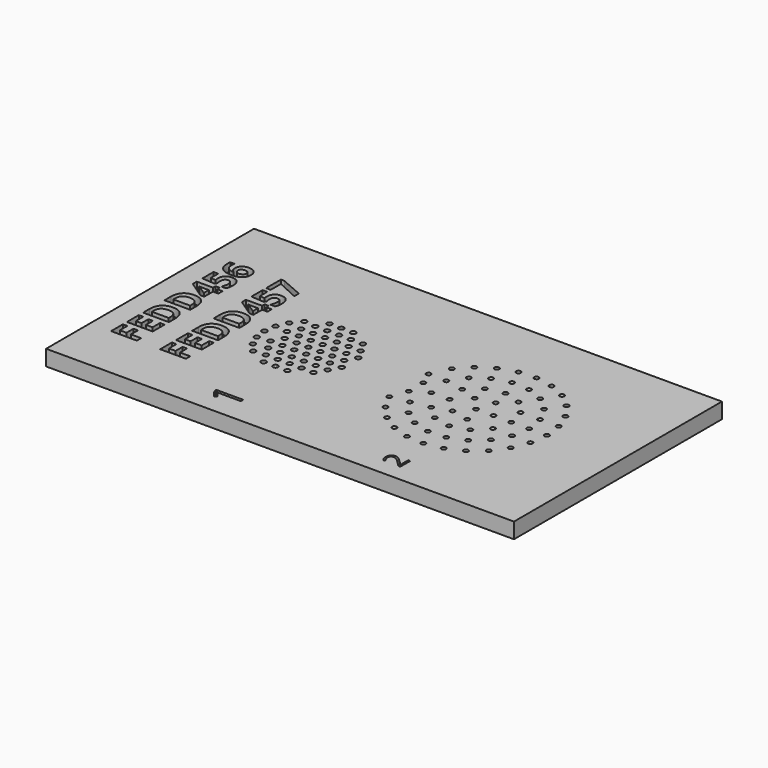
from build123d import *

# Parameters (mm, degrees)
F0_W           = 90
F0_H           = 50
F1_DEPTH       = 3
F2_TEXT_SIZE   = 6.9444444444
F2_TEXT_SIZE_2 = 7.24801812
F2_TEXT_SIZE_3 = 5.1460734388
F3_DEPTH       = 1.5
F4_R           = 0.5
F4_R_2         = 0.45
F5_DEPTH       = 3


# Not quite as in the source:
# - Text() gives the source's letters only with a copy of the font that has no kerning and outlines rounded to 1/6400 em; it was checked with that copy


with BuildPart() as f1:
    # F0 (on Top) → F1 (new body)
    with BuildSketch(Plane.XY):
        with Locations((1.8412768841, 3.3350909071)):
            Rectangle(F0_W, F0_H)
    extrude(amount=F1_DEPTH)

    # F2 (on face) → F3 (cut)
    with BuildSketch(Plane.XY.offset(3)):
        with Locations(Location((-34.1587231159, -11.7149090929), (0, 0, 90))):
            Text('FEDD456', F2_TEXT_SIZE, font='Open Sans', font_style=FontStyle.BOLD, text_align=(TextAlign.LEFT, TextAlign.BOTTOM))
        with Locations(Location((-24.7142786715, -11.7149090929), (0, 0, 90))):
            Text('FEDD457', F2_TEXT_SIZE, font='Open Sans', font_style=FontStyle.BOLD, text_align=(TextAlign.LEFT, TextAlign.BOTTOM))
        with Locations(Location((-9.6570708402, -18.6649090929), (0, 0, 90))):
            Text('1', F2_TEXT_SIZE_2, font='Open Sans', text_align=(TextAlign.LEFT, TextAlign.BOTTOM))
        with Locations(Location((22.3617675547, -18.6649090929), (0, 0, 90))):
            Text('2', F2_TEXT_SIZE_3, font='Open Sans', text_align=(TextAlign.LEFT, TextAlign.BOTTOM))
    extrude(amount=-F3_DEPTH, mode=Mode.SUBTRACT)

    # F4 (on face) → F5 (cut, through all)
    with BuildSketch(Plane.XY.offset(3)):
        with BuildLine():
            ThreePointArc((-20.6587231159, 3.3350909071), (-21.1587231159, 3.8350909071), (-21.6587231159, 3.3350909071))
            Line((-21.6587231159, 3.3350909071), (-20.6587231159, 3.3350909071))
        make_face()
        with BuildLine():
            ThreePointArc((-12.7987231159, 11.7449888556), (-13.1987231159, 11.2550909071), (-12.7987231159, 10.7651929585))
            Line((-12.7987231159, 10.7651929585), (-12.7987231159, 11.7449888556))
        make_face()
        with BuildLine():
            Line((-12.7987231159, 11.7449888556), (-12.7987231159, 10.7651929585))
            ThreePointArc((-12.7987231159, 10.7651929585), (-12.3824953499, 10.8677925724), (-12.1987231159, 11.2550909071))
            ThreePointArc((-12.1987231159, 11.2550909071), (-12.3824953499, 11.6423892417), (-12.7987231159, 11.7449888556))
        make_face()
        with BuildLine():
            ThreePointArc((-12.7987231159, 7.8049888556), (-13.1987231159, 7.3150909071), (-12.7987231159, 6.8251929585))
            Line((-12.7987231159, 6.8251929585), (-12.7987231159, 7.8049888556))
        make_face()
        with BuildLine():
            Line((-12.7987231159, 7.8049888556), (-12.7987231159, 6.8251929585))
            ThreePointArc((-12.7987231159, 6.8251929585), (-12.3824953499, 6.9277925724), (-12.1987231159, 7.3150909071))
            ThreePointArc((-12.1987231159, 7.3150909071), (-12.3824953499, 7.7023892417), (-12.7987231159, 7.8049888556))
        make_face()
        with BuildLine():
            ThreePointArc((-5.3387231159, 3.3350909071), (-5.8387231159, 3.8350909071), (-6.3387231159, 3.3350909071))
            Line((-6.3387231159, 3.3350909071), (-5.3387231159, 3.3350909071))
        make_face()
        with BuildLine():
            Line((-5.3387231159, 3.3350909071), (-6.3387231159, 3.3350909071))
            ThreePointArc((-6.3387231159, 3.3350909071), (-5.8387231159, 2.8350909071), (-5.3387231159, 3.3350909071))
        make_face()
        with BuildLine():
            ThreePointArc((-7.6287231159, 3.3350909071), (-8.1287231159, 3.8350909071), (-8.6287231159, 3.3350909071))
            Line((-8.6287231159, 3.3350909071), (-7.6287231159, 3.3350909071))
        make_face()
        with BuildLine():
            Line((-7.6287231159, 3.3350909071), (-8.6287231159, 3.3350909071))
            ThreePointArc((-8.6287231159, 3.3350909071), (-8.1287231159, 2.8350909071), (-7.6287231159, 3.3350909071))
        make_face()
        with BuildLine():
            ThreePointArc((-9.9087231159, 3.3350909071), (-10.4087231159, 3.8350909071), (-10.9087231159, 3.3350909071))
            Line((-10.9087231159, 3.3350909071), (-9.9087231159, 3.3350909071))
        make_face()
        with BuildLine():
            Line((-9.9087231159, 3.3350909071), (-10.9087231159, 3.3350909071))
            ThreePointArc((-10.9087231159, 3.3350909071), (-10.4087231159, 2.8350909071), (-9.9087231159, 3.3350909071))
        make_face()
        with BuildLine():
            ThreePointArc((-12.1987231159, -4.5849090929), (-12.3824953499, -4.1976107583), (-12.7987231159, -4.0950111444))
            Line((-12.7987231159, -4.0950111444), (-12.7987231159, -5.0748070415))
            ThreePointArc((-12.7987231159, -5.0748070415), (-12.3824953499, -4.9722074276), (-12.1987231159, -4.5849090929))
        make_face()
        with BuildLine():
            Line((-12.7987231159, -5.0748070415), (-12.7987231159, -4.0950111444))
            ThreePointArc((-12.7987231159, -4.0950111444), (-13.1987231159, -4.5849090929), (-12.7987231159, -5.0748070415))
        make_face()
        with BuildLine():
            ThreePointArc((-12.1987231159, -0.6449090929), (-12.3824953499, -0.2576107583), (-12.7987231159, -0.1550111444))
            Line((-12.7987231159, -0.1550111444), (-12.7987231159, -1.1348070415))
            ThreePointArc((-12.7987231159, -1.1348070415), (-12.3824953499, -1.0322074276), (-12.1987231159, -0.6449090929))
        make_face()
        with BuildLine():
            Line((-12.7987231159, -1.1348070415), (-12.7987231159, -0.1550111444))
            ThreePointArc((-12.7987231159, -0.1550111444), (-13.1987231159, -0.6449090929), (-12.7987231159, -1.1348070415))
        make_face()
        with BuildLine():
            ThreePointArc((-12.7987231159, 3.8249888556), (-13.0860214505, 3.6513186731), (-13.1987231159, 3.3350909071))
            Line((-13.1987231159, 3.3350909071), (-12.7987231159, 3.3350909071))
            Line((-12.7987231159, 3.3350909071), (-12.7987231159, 3.8249888556))
        make_face()
        with BuildLine():
            Line((-12.7987231159, 3.3350909071), (-13.1987231159, 3.3350909071))
            ThreePointArc((-13.1987231159, 3.3350909071), (-13.0860214505, 3.018863141), (-12.7987231159, 2.8451929585))
            Line((-12.7987231159, 2.8451929585), (-12.7987231159, 3.3350909071))
        make_face()
        with BuildLine():
            ThreePointArc((-14.4787231159, 3.3350909071), (-14.9787231159, 3.8350909071), (-15.4787231159, 3.3350909071))
            Line((-15.4787231159, 3.3350909071), (-14.4787231159, 3.3350909071))
        make_face()
        with BuildLine():
            Line((-14.4787231159, 3.3350909071), (-15.4787231159, 3.3350909071))
            ThreePointArc((-15.4787231159, 3.3350909071), (-14.9787231159, 2.8350909071), (-14.4787231159, 3.3350909071))
        make_face()
        with BuildLine():
            ThreePointArc((-16.7687231159, 3.3350909071), (-17.2687231159, 3.8350909071), (-17.7687231159, 3.3350909071))
            Line((-17.7687231159, 3.3350909071), (-16.7687231159, 3.3350909071))
        make_face()
        with BuildLine():
            Line((-16.7687231159, 3.3350909071), (-17.7687231159, 3.3350909071))
            ThreePointArc((-17.7687231159, 3.3350909071), (-17.2687231159, 2.8350909071), (-16.7687231159, 3.3350909071))
        make_face()
        with BuildLine():
            Line((-20.6587231159, 3.3350909071), (-21.6587231159, 3.3350909071))
            ThreePointArc((-21.6587231159, 3.3350909071), (-21.1587231159, 2.8350909071), (-20.6587231159, 3.3350909071))
        make_face()
        with BuildLine():
            Line((-12.7987231159, 3.8249888556), (-12.7987231159, 3.3350909071))
            Line((-12.7987231159, 3.3350909071), (-12.1987231159, 3.3350909071))
            ThreePointArc((-12.1987231159, 3.3350909071), (-12.3824953499, 3.7223892417), (-12.7987231159, 3.8249888556))
        make_face()
        with BuildLine():
            Line((-12.1987231159, 3.3350909071), (-12.7987231159, 3.3350909071))
            Line((-12.7987231159, 3.3350909071), (-12.7987231159, 2.8451929585))
            ThreePointArc((-12.7987231159, 2.8451929585), (-12.3824953499, 2.9477925724), (-12.1987231159, 3.3350909071))
        make_face()
        with Locations((-14.9787231159, -4.5849090929)):
            Circle(F4_R)
        with Locations((-18.4087231159, -2.8149090929)):
            Circle(F4_R)
        with Locations((-19.8887231159, -1.0349090929)):
            Circle(F4_R)
        with Locations((-20.8287231159, 1.0750909071)):
            Circle(F4_R)
        with Locations((-20.8287231159, 5.5950909071)):
            Circle(F4_R)
        with Locations((-19.8887231159, 7.7050909071)):
            Circle(F4_R)
        with Locations((-18.4087231159, 9.4850909071)):
            Circle(F4_R)
        with Locations((-14.9787231159, 11.2550909071)):
            Circle(F4_R)
        with Locations((-10.4087231159, 11.2550909071)):
            Circle(F4_R)
        with Locations((-6.9787231159, 9.2750909071)):
            Circle(F4_R)
        with Locations((-5.8387231159, 7.2950909071)):
            Circle(F4_R)
        with Locations((-4.6987231159, 5.3150909071)):
            Circle(F4_R)
        with Locations((-4.6987231159, 1.3550909071)):
            Circle(F4_R)
        with Locations((-5.8387231159, -0.6249090929)):
            Circle(F4_R)
        with Locations((-6.9787231159, -2.6049090929)):
            Circle(F4_R)
        with Locations((-10.4087231159, -4.5849090929)):
            Circle(F4_R)
        with Locations((-18.4087231159, 5.3150909071)):
            Circle(F4_R)
        with Locations((-17.2687231159, 7.2950909071)):
            Circle(F4_R)
        with Locations((-16.1287231159, 9.2750909071)):
            Circle(F4_R)
        with Locations((-13.8387231159, 9.2750909071)):
            Circle(F4_R)
        with Locations((-16.1287231159, 5.3150909071)):
            Circle(F4_R)
        with Locations((-14.9787231159, 7.2950909071)):
            Circle(F4_R)
        with Locations((-13.8387231159, 5.3150909071)):
            Circle(F4_R)
        with Locations((-9.2687231159, 9.2750909071)):
            Circle(F4_R)
        with Locations((-8.1287231159, 7.2950909071)):
            Circle(F4_R)
        with Locations((-9.2687231159, 5.3150909071)):
            Circle(F4_R)
        with Locations((-10.4087231159, 7.2950909071)):
            Circle(F4_R)
        with Locations((-11.5587231159, 5.3150909071)):
            Circle(F4_R)
        with Locations((-18.4087231159, 1.3550909071)):
            Circle(F4_R)
        with Locations((-16.1287231159, 1.3550909071)):
            Circle(F4_R)
        with Locations((-13.8387231159, 1.3550909071)):
            Circle(F4_R)
        with Locations((-11.5587231159, 1.3550909071)):
            Circle(F4_R)
        with Locations((-9.2687231159, 1.3550909071)):
            Circle(F4_R)
        with Locations((-6.9787231159, 1.3550909071)):
            Circle(F4_R)
        with Locations((-17.2687231159, -0.6249090929)):
            Circle(F4_R)
        with Locations((-14.9787231159, -0.6249090929)):
            Circle(F4_R)
        with Locations((-10.4087231159, -0.6249090929)):
            Circle(F4_R)
        with Locations((-8.1287231159, -0.6249090929)):
            Circle(F4_R)
        with Locations((-16.1287231159, -2.6049090929)):
            Circle(F4_R)
        with Locations((-13.8387231159, -2.6049090929)):
            Circle(F4_R)
        with Locations((-11.5587231159, -2.6049090929)):
            Circle(F4_R)
        with Locations((-9.2687231159, -2.6049090929)):
            Circle(F4_R)
        with Locations((-6.9787231159, 5.3150909071)):
            Circle(F4_R)
        with Locations((-11.5587231159, 9.2750909071)):
            Circle(F4_R)
        with BuildLine():
            ThreePointArc((11.4012768841, 3.3350909071), (10.9512768841, 3.7850909071), (10.5012768841, 3.3350909071))
            Line((10.5012768841, 3.3350909071), (11.4012768841, 3.3350909071))
        make_face()
        with BuildLine():
            ThreePointArc((19.5412768841, 10.4892566457), (19.3412768841, 10.1150909071), (19.5412768841, 9.7409251684))
            Line((19.5412768841, 9.7409251684), (19.5412768841, 10.4892566457))
        make_face()
        with BuildLine():
            Line((19.5412768841, 10.4892566457), (19.5412768841, 9.7409251684))
            ThreePointArc((19.5412768841, 9.7409251684), (20.0034089184, 9.7182282104), (20.2412768841, 10.1150909071))
            ThreePointArc((20.2412768841, 10.1150909071), (20.0034089184, 10.5119536037), (19.5412768841, 10.4892566457))
        make_face()
        with BuildLine():
            ThreePointArc((33.6312768841, 3.3350909071), (33.1812768841, 3.7850909071), (32.7312768841, 3.3350909071))
            Line((32.7312768841, 3.3350909071), (33.6312768841, 3.3350909071))
        make_face()
        with BuildLine():
            Line((33.6312768841, 3.3350909071), (32.7312768841, 3.3350909071))
            ThreePointArc((32.7312768841, 3.3350909071), (33.1812768841, 2.8850909071), (33.6312768841, 3.3350909071))
        make_face()
        with BuildLine():
            ThreePointArc((30.2012768841, 3.3350909071), (29.7512768841, 3.7850909071), (29.3012768841, 3.3350909071))
            Line((29.3012768841, 3.3350909071), (30.2012768841, 3.3350909071))
        make_face()
        with BuildLine():
            Line((30.2012768841, 3.3350909071), (29.3012768841, 3.3350909071))
            ThreePointArc((29.3012768841, 3.3350909071), (29.7512768841, 2.8850909071), (30.2012768841, 3.3350909071))
        make_face()
        with BuildLine():
            ThreePointArc((26.7712768841, 3.3350909071), (26.3212768841, 3.7850909071), (25.8712768841, 3.3350909071))
            Line((25.8712768841, 3.3350909071), (26.7712768841, 3.3350909071))
        make_face()
        with BuildLine():
            Line((26.7712768841, 3.3350909071), (25.8712768841, 3.3350909071))
            ThreePointArc((25.8712768841, 3.3350909071), (26.3212768841, 2.8850909071), (26.7712768841, 3.3350909071))
        make_face()
        with BuildLine():
            ThreePointArc((23.3412768841, 3.3350909071), (22.8912768841, 3.7850909071), (22.4412768841, 3.3350909071))
            Line((22.4412768841, 3.3350909071), (23.3412768841, 3.3350909071))
        make_face()
        with BuildLine():
            Line((23.3412768841, 3.3350909071), (22.4412768841, 3.3350909071))
            ThreePointArc((22.4412768841, 3.3350909071), (22.8912768841, 2.8850909071), (23.3412768841, 3.3350909071))
        make_face()
        with BuildLine():
            ThreePointArc((20.2412768841, -3.4449090929), (20.0034089184, -3.0480463963), (19.5412768841, -3.0707433543))
            Line((19.5412768841, -3.0707433543), (19.5412768841, -3.8190748316))
            ThreePointArc((19.5412768841, -3.8190748316), (20.0034089184, -3.8417717896), (20.2412768841, -3.4449090929))
        make_face()
        with BuildLine():
            Line((19.5412768841, -3.8190748316), (19.5412768841, -3.0707433543))
            ThreePointArc((19.5412768841, -3.0707433543), (19.3412768841, -3.4449090929), (19.5412768841, -3.8190748316))
        make_face()
        with BuildLine():
            ThreePointArc((19.5412768841, 3.7850909071), (19.2230788325, 3.6532889586), (19.0912768841, 3.3350909071))
            Line((19.0912768841, 3.3350909071), (19.5412768841, 3.3350909071))
            Line((19.5412768841, 3.3350909071), (19.5412768841, 3.7850909071))
        make_face()
        with BuildLine():
            Line((19.5412768841, 3.3350909071), (19.0912768841, 3.3350909071))
            ThreePointArc((19.0912768841, 3.3350909071), (19.2230788325, 3.0168928555), (19.5412768841, 2.8850909071))
            Line((19.5412768841, 2.8850909071), (19.5412768841, 3.3350909071))
        make_face()
        with BuildLine():
            ThreePointArc((14.9112768841, 3.3350909071), (14.4612768841, 3.7850909071), (14.0112768841, 3.3350909071))
            Line((14.0112768841, 3.3350909071), (14.9112768841, 3.3350909071))
        make_face()
        with BuildLine():
            Line((14.9112768841, 3.3350909071), (14.0112768841, 3.3350909071))
            ThreePointArc((14.0112768841, 3.3350909071), (14.4612768841, 2.8850909071), (14.9112768841, 3.3350909071))
        make_face()
        with BuildLine():
            Line((11.4012768841, 3.3350909071), (10.5012768841, 3.3350909071))
            ThreePointArc((10.5012768841, 3.3350909071), (10.9512768841, 2.8850909071), (11.4012768841, 3.3350909071))
        make_face()
        with BuildLine():
            Line((19.5412768841, 3.7850909071), (19.5412768841, 3.3350909071))
            Line((19.5412768841, 3.3350909071), (19.9912768841, 3.3350909071))
            ThreePointArc((19.9912768841, 3.3350909071), (19.8594749356, 3.6532889586), (19.5412768841, 3.7850909071))
        make_face()
        with BuildLine():
            Line((19.9912768841, 3.3350909071), (19.5412768841, 3.3350909071))
            Line((19.5412768841, 3.3350909071), (19.5412768841, 2.8850909071))
            ThreePointArc((19.5412768841, 2.8850909071), (19.8594749356, 3.0168928555), (19.9912768841, 3.3350909071))
        make_face()
        with Locations((6.8412768841, 7.8150909071)):
            Circle(F4_R_2)
        with Locations((8.4912768841, 11.3150909071)):
            Circle(F4_R_2)
        with Locations((10.8312768841, 13.8250909071)):
            Circle(F4_R_2)
        with Locations((13.7012768841, 15.6550909071)):
            Circle(F4_R_2)
        with Locations((16.9712768841, 16.7250909071)):
            Circle(F4_R_2)
        with Locations((20.3012768841, 16.9450909071)):
            Circle(F4_R_2)
        with Locations((23.7112768841, 16.3150909071)):
            Circle(F4_R_2)
        with Locations((26.8312768841, 14.8650909071)):
            Circle(F4_R_2)
        with Locations((29.4712768841, 12.6850909071)):
            Circle(F4_R_2)
        with Locations((31.4812768841, 9.9150909071)):
            Circle(F4_R_2)
        with Locations((32.7212768841, 6.7350909071)):
            Circle(F4_R_2)
        with Locations((32.7212768841, -0.0649090929)):
            Circle(F4_R_2)
        with Locations((31.4812768841, -3.2449090929)):
            Circle(F4_R_2)
        with Locations((29.4712768841, -6.0149090929)):
            Circle(F4_R_2)
        with Locations((26.8312768841, -8.1949090929)):
            Circle(F4_R_2)
        with Locations((23.7112768841, -9.6449090929)):
            Circle(F4_R_2)
        with Locations((20.3012768841, -10.2749090929)):
            Circle(F4_R_2)
        with Locations((16.9712768841, -10.0549090929)):
            Circle(F4_R_2)
        with Locations((13.7012768841, -8.9849090929)):
            Circle(F4_R_2)
        with Locations((10.8312768841, -7.1549090929)):
            Circle(F4_R_2)
        with Locations((8.4912768841, -4.6449090929)):
            Circle(F4_R_2)
        with Locations((6.8412768841, -1.6449090929)):
            Circle(F4_R_2)
        with Locations((8.0112768841, 5.0650909071)):
            Circle(F4_R_2)
        with Locations((10.3212768841, 7.7250909071)):
            Circle(F4_R_2)
        with Locations((12.3512768841, 10.5750909071)):
            Circle(F4_R_2)
        with Locations((15.0912768841, 12.5250909071)):
            Circle(F4_R_2)
        with Locations((18.3712768841, 13.4650909071)):
            Circle(F4_R_2)
        with Locations((21.7812768841, 13.2950909071)):
            Circle(F4_R_2)
        with Locations((24.9512768841, 11.9950909071)):
            Circle(F4_R_2)
        with Locations((27.5212768841, 9.7150909071)):
            Circle(F4_R_2)
        with Locations((23.0712768841, 9.1250909071)):
            Circle(F4_R_2)
        with Locations((25.4612768841, 6.6650909071)):
            Circle(F4_R_2)
        with Locations((20.5812768841, 6.7650909071)):
            Circle(F4_R_2)
        with Locations((13.8812768841, 7.0650909071)):
            Circle(F4_R_2)
        with Locations((16.4412768841, 9.3550909071)):
            Circle(F4_R_2)
        with Locations((17.1512768841, 6.0050909071)):
            Circle(F4_R_2)
        with Locations((8.0112768841, 1.6050909071)):
            Circle(F4_R_2)
        with Locations((10.3212768841, -1.0549090929)):
            Circle(F4_R_2)
        with Locations((12.3512768841, -3.9049090929)):
            Circle(F4_R_2)
        with Locations((15.0912768841, -5.8549090929)):
            Circle(F4_R_2)
        with Locations((18.3712768841, -6.7949090929)):
            Circle(F4_R_2)
        with Locations((13.8812768841, -0.3949090929)):
            Circle(F4_R_2)
        with Locations((16.4412768841, -2.6849090929)):
            Circle(F4_R_2)
        with Locations((17.1512768841, 0.6650909071)):
            Circle(F4_R_2)
        with Locations((25.4612768841, 0.0050909071)):
            Circle(F4_R_2)
        with Locations((29.1712768841, -0.0449090929)):
            Circle(F4_R_2)
        with Locations((27.5212768841, -3.0449090929)):
            Circle(F4_R_2)
        with Locations((24.9512768841, -5.3149090929)):
            Circle(F4_R_2)
        with Locations((21.7812768841, -6.6249090929)):
            Circle(F4_R_2)
        with Locations((20.5812768841, -0.0949090929)):
            Circle(F4_R_2)
        with Locations((29.1712768841, 6.7150909071)):
            Circle(F4_R_2)
        with Locations((23.0712768841, -2.4549090929)):
            Circle(F4_R_2)
    extrude(amount=-F5_DEPTH, mode=Mode.SUBTRACT)


solid = f1.part
